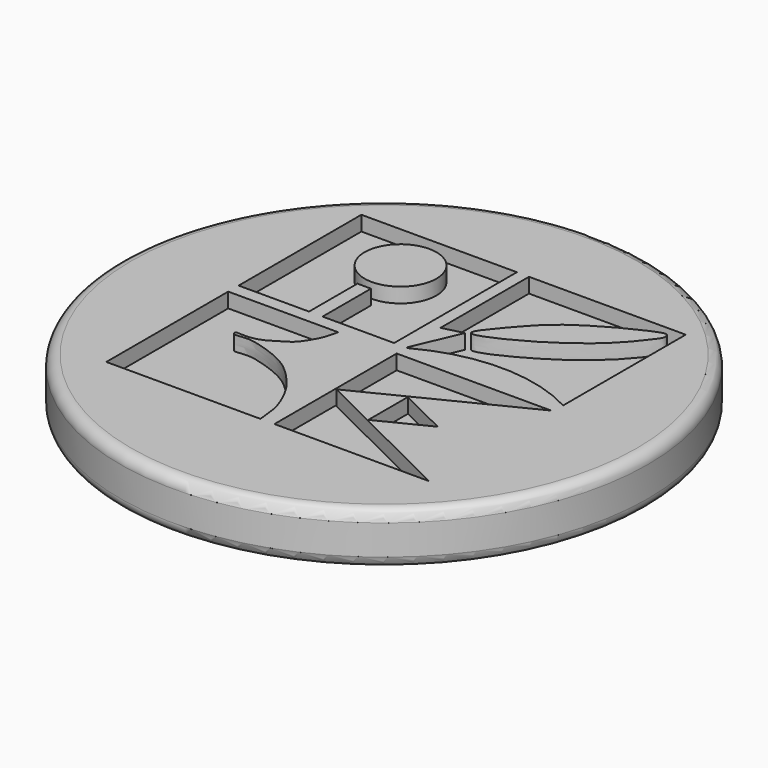
from build123d import *

# Parameters (mm, degrees)
F1_R      = 12.125
F1_W      = 7.0986367516
F1_H      = 7.0182182118
F2_DEPTH  = 2.38
F3_R      = 0.5
F4_R      = 0.5
F1_W_2    = 0.6225926336
F1_H_2    = 2.7800722164
F1_R_2    = 1.6491882735
F5_DEPTH  = 1.7
F6_DEPTH  = 2.38
F7_DEPTH  = 1.7
F8_DEPTH  = 2.38
F9_DEPTH  = 1.7
F10_DEPTH = 2.38
F11_DEPTH = 1.7
F12_DEPTH = 2.38


# Not quite as in the source:
# - a feature names something its author has since deleted; it is built from what else it names


with BuildPart() as f2:
    # F1 (on Top) → F2 (new body)
    with BuildSketch(Plane.XY):
        Circle(F1_R)
        Polygon((-7.4228290468, -6.6703339335), (-7.4228290468, 0.3279154543), (-2.3676725104, 0.3279154543), (-0.2785333199, 0.3279154543), (-0.2785333199, -6.6703339335), (-0.3460554872, -6.6703339335), align=None, mode=Mode.SUBTRACT)
        with Locations((3.8493661203, -3.1612248276)):
            Rectangle(F1_W, F1_H, mode=Mode.SUBTRACT)
        Polygon((-7.4221123941, 0.9262498352), (-7.4221123941, 7.9733738676), (-0.2785333199, 7.9733738676), (-0.2785333199, 0.9262498352), (-3.5664748866, 0.9262498352), (-4.1890675202, 0.9262498352), align=None, mode=Mode.SUBTRACT)
        Polygon((0.2827075659, 2.8855106793), (0.2827075659, 7.9663181677), (7.483521942, 7.9663181677), (7.483521942, 0.9262498352), (0.3603694204, 0.9262498352), (0.2827075659, 0.9262498352), align=None, mode=Mode.SUBTRACT)
    extrude(amount=F2_DEPTH)

    # F3
    f3_edges = [f2.edges().sort_by_distance(p)[0] for p in [
        (-12.125, 0, 2.38),
    ]]
    fillet(f3_edges, radius=F3_R)

    # F4
    f4_edges = [f2.edges().sort_by_distance(p)[0] for p in [
        (-12.125, 0, 0),
    ]]
    fillet(f4_edges, radius=F4_R)

    # F1 (on Top) → F5 (join)
    with BuildSketch(Plane.XY):
        with Locations((-3.8777712034, 2.3162859434)):
            Rectangle(F1_W_2, F1_H_2)
        Polygon((-0.2785333199, 7.9733738676), (-7.4221123941, 7.9733738676), (-7.4221123941, 0.9262498352), (-4.1890675202, 0.9262498352), (-4.1890675202, 3.7063220516), (-3.5664748866, 3.7063220516), (-3.5664748866, 0.9262498352), (-0.2785333199, 0.9262498352), align=None)
        with Locations((-3.8649578562, 5.7759984099)):
            Circle(F1_R_2, mode=Mode.SUBTRACT)
        with Locations((-3.8649578562, 5.7759984099)):
            Circle(F1_R_2)
    extrude(amount=F5_DEPTH)

    # F1 (on Top) → F6 (join, through all)
    with BuildSketch(Plane.XY):
        with Locations((-3.8649578562, 5.7759984099)):
            Circle(F1_R_2)
        with Locations((-3.8777712034, 2.3162859434)):
            Rectangle(F1_W_2, F1_H_2)
    extrude(amount=F6_DEPTH)

    # F1 (on Top) → F7 (join)
    with BuildSketch(Plane.XY):
        Polygon((7.3986844961, 0.3478842783), (0.3000477445, 0.3478842783), (0.3000477445, -6.6703339335), (7.3986844961, -6.6703339335), (0.3533055715, -3.1787578482), align=None)
        Polygon((7.3986844961, -6.6703339335), (7.3986844961, 0.3478842783), (0.3533055715, -3.1787578482), align=None)
        Polygon((2.7262428775, -4.3149543926), (2.7262428775, -2.0406346302), (5.0051301037, -3.174232257), align=None, mode=Mode.SUBTRACT)
        Polygon((5.0051301037, -3.174232257), (2.7262428775, -2.0406346302), (2.7262428775, -4.3149543926), align=None)
    extrude(amount=F7_DEPTH)

    # F1 (on Top) → F8 (join, through all)
    with BuildSketch(Plane.XY):
        Polygon((7.3986844961, -6.6703339335), (7.3986844961, 0.3478842783), (0.3533055715, -3.1787578482), align=None)
        Polygon((2.7262428775, -4.3149543926), (2.7262428775, -2.0406346302), (5.0051301037, -3.174232257), align=None, mode=Mode.SUBTRACT)
    extrude(amount=F8_DEPTH)

    # F1 (on Top) → F9 (join)
    with BuildSketch(Plane.XY):
        with BuildLine():
            Line((7.483521942, 7.9663181677), (0.2827075659, 7.9663181677))
            Line((0.2827075659, 7.9663181677), (0.2827075659, 2.8855106793))
            Line((0.2827075659, 2.8855106793), (1.2191495625, 3.121049609))
            Line((1.2191495625, 3.121049609), (0.2827075659, 0.9262498352))
            Line((0.2827075659, 0.9262498352), (0.3603694204, 0.9262498352))
            ThreePointArc((0.3603694204, 0.9262498352), (3.9219456812, 1.8291393853), (7.483521942, 0.9262498352))
            Line((7.483521942, 0.9262498352), (7.483521942, 7.9663181677))
        make_face()
        with BuildLine():
            add(Edge.make_bspline(
                [(1.3767119963, 3.2667766791), (1.2845749547, 3.4219093882), (2.4235264698, 4.7283232609), (3.5408753586, 5.9956475692), (6.2391393141, 7.418797197), (6.8917216898, 7.5995638626), (6.9665371868, 7.5324135615), (7.0858412946, 7.3423232683), (6.6731021166, 6.7922406039), (5.7276068284, 5.5974675028), (3.4869356373, 3.9709181084), (1.4800923213, 3.0927134618), (1.3767119963, 3.2667766791)],
                knots=[0, 0, 0, 0, 0.1118483914, 0.24448623, 0.4022164571, 0.4698846563, 0.4939539155, 0.5310056289, 0.6004556126, 0.7122838549, 0.8745029919, 1, 1, 1, 1], degree=3))
        make_face(mode=Mode.SUBTRACT)
        with BuildLine():
            add(Edge.make_bspline(
                [(1.3767119963, 3.2667766791), (1.2845749547, 3.4219093882), (2.4235264698, 4.7283232609), (3.5408753586, 5.9956475692), (6.2391393141, 7.418797197), (6.8917216898, 7.5995638626), (6.9665371868, 7.5324135615), (7.0858412946, 7.3423232683), (6.6731021166, 6.7922406039), (5.7276068284, 5.5974675028), (3.4869356373, 3.9709181084), (1.4800923213, 3.0927134618), (1.3767119963, 3.2667766791)],
                knots=[0, 0, 0, 0, 0.1118483914, 0.24448623, 0.4022164571, 0.4698846563, 0.4939539155, 0.5310056289, 0.6004556126, 0.7122838549, 0.8745029919, 1, 1, 1, 1], degree=3))
        make_face()
        with BuildLine():
            Line((0.3603694204, 0.9262498352), (7.483521942, 0.9262498352))
            ThreePointArc((7.483521942, 0.9262498352), (3.9219456812, 1.8291393853), (0.3603694204, 0.9262498352))
        make_face()
        Polygon((1.2191495625, 3.121049609), (0.2827075659, 2.8855106793), (0.2827075659, 0.9262498352), align=None)
    extrude(amount=F9_DEPTH)

    # F1 (on Top) → F10 (join, through all)
    with BuildSketch(Plane.XY):
        Polygon((1.2191495625, 3.121049609), (0.2827075659, 2.8855106793), (0.2827075659, 0.9262498352), align=None)
        with BuildLine():
            Line((0.3603694204, 0.9262498352), (7.483521942, 0.9262498352))
            ThreePointArc((7.483521942, 0.9262498352), (3.9219456812, 1.8291393853), (0.3603694204, 0.9262498352))
        make_face()
        with BuildLine():
            add(Edge.make_bspline(
                [(1.3767119963, 3.2667766791), (1.2845749547, 3.4219093882), (2.4235264698, 4.7283232609), (3.5408753586, 5.9956475692), (6.2391393141, 7.418797197), (6.8917216898, 7.5995638626), (6.9665371868, 7.5324135615), (7.0858412946, 7.3423232683), (6.6731021166, 6.7922406039), (5.7276068284, 5.5974675028), (3.4869356373, 3.9709181084), (1.4800923213, 3.0927134618), (1.3767119963, 3.2667766791)],
                knots=[0, 0, 0, 0, 0.1118483914, 0.24448623, 0.4022164571, 0.4698846563, 0.4939539155, 0.5310056289, 0.6004556126, 0.7122838549, 0.8745029919, 1, 1, 1, 1], degree=3))
        make_face()
    extrude(amount=F10_DEPTH)

    # F1 (on Top) → F11 (join)
    with BuildSketch(Plane.XY):
        with BuildLine():
            Line((-2.3676725104, 0.3279154543), (-7.4228290468, 0.3279154543))
            Line((-7.4228290468, 0.3279154543), (-7.4228290468, -6.6703339335))
            Line((-7.4228290468, -6.6703339335), (-0.3460554872, -6.6703339335))
            add(Edge.make_bspline(
                [(-2.3676725104, 0.3279154543), (-2.4010776229, 0.1925208975), (-2.4676626782, -0.0773555796), (-2.5876283556, -0.4592288495), (-2.8925989526, -0.9591658513), (-3.1522335022, -1.2984425332), (-3.7077309843, -1.5983279611), (-3.9910833592, -1.8042724956), (-4.6138242999, -2.0322850474), (-5.2750707973, -1.9267077545), (-5.2495717166, -2.0402242976), (-5.2345405936, -2.0988768979), (-5.1450714886, -2.160796158), (-4.6968573849, -2.0831274685), (-4.1628510391, -2.1198506981), (-2.7612179261, -2.5768069629), (-1.9266213932, -3.2203760963), (-1.1791410617, -4.0827112095), (-0.8290586767, -4.6976898082), (-0.4695580442, -5.5403229192), (-0.4210791981, -6.0329268408), (-0.3569856889, -6.488706617), (-0.3490962485, -6.6198055594), (-0.3460554872, -6.6703339335)],
                knots=[0, 0, 0, 0, 0.0435833884, 0.086873, 0.1381261489, 0.1834527151, 0.2360140714, 0.2766814959, 0.3332809415, 0.3847393962, 0.400679245, 0.417088421, 0.4369598891, 0.4804923093, 0.5317269995, 0.6128329106, 0.6846024733, 0.7554901569, 0.8138428178, 0.8776633918, 0.9266412888, 0.9717259625, 1, 1, 1, 1], degree=3))
        make_face()
        with BuildLine():
            Line((-0.2785333199, 0.3279154543), (-2.3676725104, 0.3279154543))
            add(Edge.make_bspline(
                [(-2.3676725104, 0.3279154543), (-2.4010776229, 0.1925208975), (-2.4676626782, -0.0773555796), (-2.5876283556, -0.4592288495), (-2.8925989526, -0.9591658513), (-3.1522335022, -1.2984425332), (-3.7077309843, -1.5983279611), (-3.9910833592, -1.8042724956), (-4.6138242999, -2.0322850474), (-5.2750707973, -1.9267077545), (-5.2495717166, -2.0402242976), (-5.2345405936, -2.0988768979), (-5.1450714886, -2.160796158), (-4.6968573849, -2.0831274685), (-4.1628510391, -2.1198506981), (-2.7612179261, -2.5768069629), (-1.9266213932, -3.2203760963), (-1.1791410617, -4.0827112095), (-0.8290586767, -4.6976898082), (-0.4695580442, -5.5403229192), (-0.4210791981, -6.0329268408), (-0.3569856889, -6.488706617), (-0.3490962485, -6.6198055594), (-0.3460554872, -6.6703339335)],
                knots=[0, 0, 0, 0, 0.0435833884, 0.086873, 0.1381261489, 0.1834527151, 0.2360140714, 0.2766814959, 0.3332809415, 0.3847393962, 0.400679245, 0.417088421, 0.4369598891, 0.4804923093, 0.5317269995, 0.6128329106, 0.6846024733, 0.7554901569, 0.8138428178, 0.8776633918, 0.9266412888, 0.9717259625, 1, 1, 1, 1], degree=3))
            Line((-0.3460554872, -6.6703339335), (-0.2785333199, -6.6703339335))
            Line((-0.2785333199, -6.6703339335), (-0.2785333199, 0.3279154543))
        make_face()
    extrude(amount=F11_DEPTH)

    # F1 (on Top) → F12 (join, through all)
    with BuildSketch(Plane.XY):
        with BuildLine():
            Line((-0.2785333199, 0.3279154543), (-2.3676725104, 0.3279154543))
            add(Edge.make_bspline(
                [(-2.3676725104, 0.3279154543), (-2.4010776229, 0.1925208975), (-2.4676626782, -0.0773555796), (-2.5876283556, -0.4592288495), (-2.8925989526, -0.9591658513), (-3.1522335022, -1.2984425332), (-3.7077309843, -1.5983279611), (-3.9910833592, -1.8042724956), (-4.6138242999, -2.0322850474), (-5.2750707973, -1.9267077545), (-5.2495717166, -2.0402242976), (-5.2345405936, -2.0988768979), (-5.1450714886, -2.160796158), (-4.6968573849, -2.0831274685), (-4.1628510391, -2.1198506981), (-2.7612179261, -2.5768069629), (-1.9266213932, -3.2203760963), (-1.1791410617, -4.0827112095), (-0.8290586767, -4.6976898082), (-0.4695580442, -5.5403229192), (-0.4210791981, -6.0329268408), (-0.3569856889, -6.488706617), (-0.3490962485, -6.6198055594), (-0.3460554872, -6.6703339335)],
                knots=[0, 0, 0, 0, 0.0435833884, 0.086873, 0.1381261489, 0.1834527151, 0.2360140714, 0.2766814959, 0.3332809415, 0.3847393962, 0.400679245, 0.417088421, 0.4369598891, 0.4804923093, 0.5317269995, 0.6128329106, 0.6846024733, 0.7554901569, 0.8138428178, 0.8776633918, 0.9266412888, 0.9717259625, 1, 1, 1, 1], degree=3))
            Line((-0.3460554872, -6.6703339335), (-0.2785333199, -6.6703339335))
            Line((-0.2785333199, -6.6703339335), (-0.2785333199, 0.3279154543))
        make_face()
    extrude(amount=F12_DEPTH)


solid = f2.part
